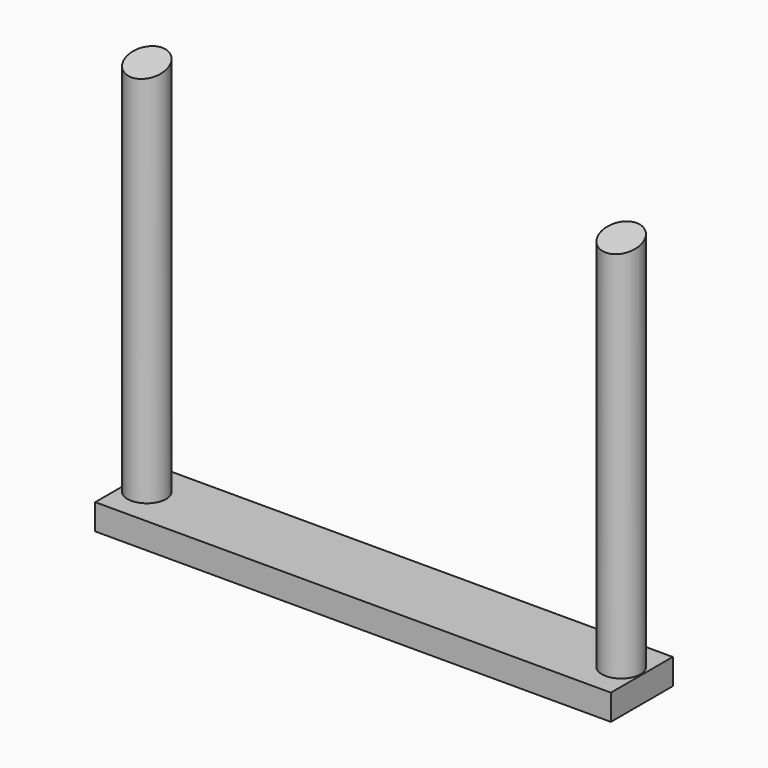
from build123d import *

# Parameters (mm, degrees)
F0_W          = 50.8
F0_H          = 7.62
F1_DEPTH      = 2.54
F2_R          = 1.905
F3_DEPTH      = 38.1
F5_DEPTH      = 50.801
F5_DEPTH_BACK = 94


# Not quite as in the source:
# - an extrude ends at something that could not be found from the text; its depth is read off the source's solid


with BuildPart() as f1:
    # F0 (on Top) → F1 (new body)
    with BuildSketch(Plane.XY):
        with Locations((25.4, 3.81)):
            Rectangle(F0_W, F0_H)
    extrude(amount=F1_DEPTH)

    # F2 (on face) → F3 (join)
    with BuildSketch(Plane.XY.offset(2.54)):
        with Locations((2.032, 3.81)):
            Circle(F2_R)
        with Locations((48.768, 3.81)):
            Circle(F2_R)
    extrude(amount=F3_DEPTH)

    # F4 (on Right) → F5 (cut, two sides)
    with BuildSketch(Plane.YZ) as f5_sk:
        Polygon((0, 40.64), (0, 38.7614695235), (7.5709112298, 40.7900890735), align=None)
    extrude(amount=F5_DEPTH, mode=Mode.SUBTRACT)
    extrude(f5_sk.sketch, amount=-F5_DEPTH_BACK, mode=Mode.SUBTRACT)


solid = f1.part
